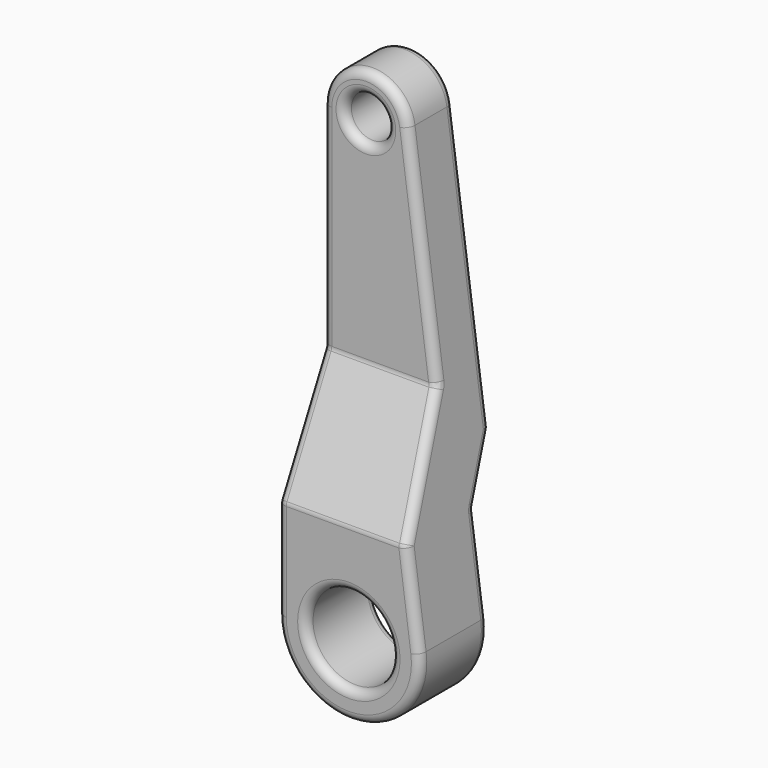
from build123d import *

# Parameters (mm, degrees)
F1_DEPTH = 40
F2_W     = 20
F2_H     = 15.9666295471
F2_W_2   = 10
F2_H_2   = 25.9443825785
F3_DEPTH = 50.001
F4_R     = 7.5
F4_R_2   = 15
F5_DEPTH = 40.001
F6_T     = -8
F8_DEPTH = 14
F9_R     = 3


with BuildPart() as f1:
    # F0 (on Front) → F1 (new body)
    with BuildSketch(Plane.XZ):
        with BuildLine():
            Line((-25, 149.666295471), (-25, 0))
            ThreePointArc((-25, 0), (1.6666666667, -24.9443825785), (24.7777777778, 3.3259176771))
            Line((24.7777777778, 3.3259176771), (4.8666666667, 151.6618460772))
            ThreePointArc((4.8666666667, 151.6618460772), (-11, 164.6329250181), (-25, 149.666295471))
        make_face()
    extrude(amount=F1_DEPTH)

    # F2 (on face) → F3 (cut, through all)
    with BuildSketch(Plane(origin=(-25, 0, 0), x_dir=(0, -1, 0), z_dir=(-1, 0, 0))):
        Polygon((40, 149.666295471), (20, 149.666295471), (20, 75), (40, 35), align=None)
        with Locations((30, 157.6496102445)):
            Rectangle(F2_W, F2_H)
        Polygon((0, 55), (0, 0), (10, 0), (10, 35), align=None)
        with Locations((5, -12.9721912892)):
            Rectangle(F2_W_2, F2_H_2)
    extrude(amount=-F3_DEPTH, mode=Mode.SUBTRACT)

    # F4 (on face) → F5 (cut, through all)
    with BuildSketch(Plane(origin=(0, 0, 0), x_dir=(-1, 0, 0), z_dir=(0, 1, 0))):
        with Locations((10, 149.666295471)):
            Circle(F4_R)
        Circle(F4_R_2)
    extrude(amount=-F5_DEPTH, mode=Mode.SUBTRACT)

    # F6
    f6_openings = [f1.faces().sort_by_distance(p)[0] for p in [
        (-6.738157, 0, 102.644086),
        (-2.901268, -5.050633, 44.898734),
        (-24.218975, -10, 17.5),
    ]]
    offset(amount=F6_T, openings=f6_openings)

    # F7 (on face) → F8 (join, through all)
    with BuildSketch(Plane(origin=(0, 0, 0), x_dir=(-1, 0, 0), z_dir=(0, 1, 0))):
        Polygon((17, 77.11145618), (-6.8018062916, 77.11145618), (-7.8756451829, 69.11145618), (17, 69.11145618), align=None)
    extrude(amount=-F8_DEPTH)

    # F9
    f9_edges = [f1.edges().sort_by_distance(p)[0] for p in [
        (-21, 0, 55),
        (-25, -5, 45),
        (-21, -10, 35),
        (-17, -5, 45),
        (16.490296, -10, 35),
        (19.183871, -5, 45),
        (13.805698, 0, 55),
        (11.112123, -5, 45),
        (-17, -23, 51.111456),
        (-2.14604, -32, 33.111456),
        (10.291783, -23, 51.111456),
        (-4.562177, -14, 69.111456),
        (-17, 0, 62.055728),
        (-17, -10, 25.245967),
        (-17, -21, 15.491933),
        (-17, -32, 24.301695),
        (-17, -7, 69.111456),
        (13.621157, -10, 26.307926),
        (8.822735, 0, 62.055728),
        (7.875645, -7, 69.111456),
        (13.747907, -32, 25.363654),
        (14.787893, -21, 17.615851),
        (-25, -10, 17.5),
        (1.666667, -10, -24.944383),
        (22.651974, -10, 19.162959),
        (-1.533333, -10, 22.948832),
        (15, -10, 0),
        (-25, -30, 55),
        (-2.236915, -40, 35),
        (17.841573, -30, 55),
        (-4.921512, -20, 75),
        (-25, -40, 17.5),
        (22.651974, -40, 19.162959),
        (1.666667, -40, -24.944383),
        (15, -40, 0),
        (2.789695, 0, 107.00131),
        (-1.222415, -6, 136.891163),
        (2.789695, -12, 107.00131),
        (6.801806, -6, 77.111456),
        (-25, -20, 112.333148),
        (-11, -20, 164.632925),
        (10.011821, -20, 113.330923),
        (-2.5, -20, 149.666295),
        (-2.5, 0, 149.666295),
        (-17.5, -10, 149.666295),
        (-5.099097, -12, 77.111456),
        (-8.966667, -12, 134.200778),
        (-17, -12, 106.474217),
        (-8.966667, 0, 134.200778),
        (-17, -6, 135.836979),
        (-5.099097, 0, 77.111456),
        (11.35412, 0, 103.330923),
        (4.866667, -10, 151.661846),
        (24.777778, -25, 3.325918),
        (-25, 0, 102.333148),
        (-4.562177, 0, 69.111456),
        (-11, 0, 164.632925),
        (-17, -6, 77.111456),
        (-17, 0, 106.474217),
    ]]
    fillet(f9_edges, radius=F9_R)


solid = f1.part
